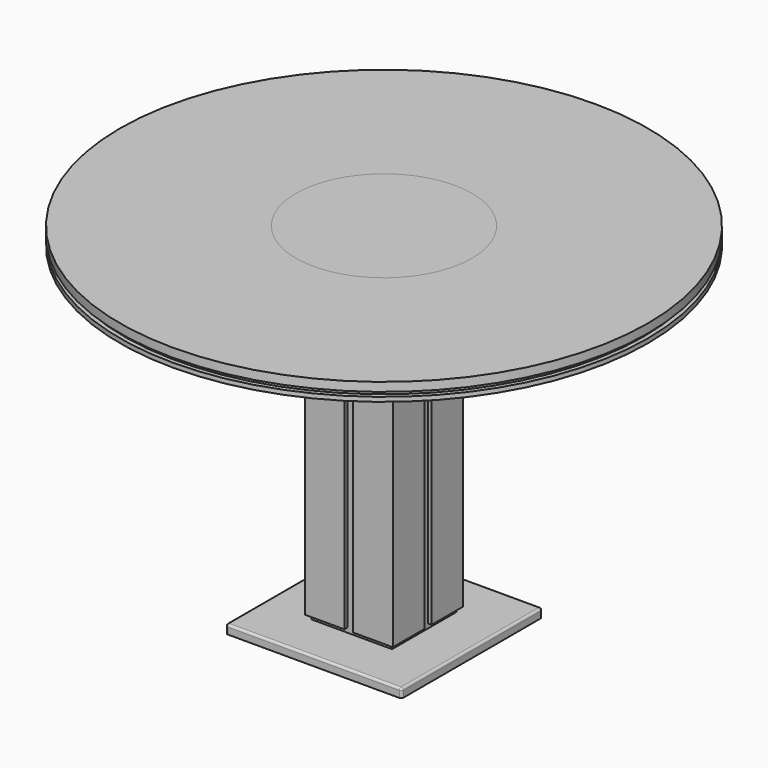
from build123d import *

# Parameters (mm, degrees)
F1_START  = 30
F1_DEPTH  = 720
F2_START  = 30
F0_W      = 20
F0_H      = 8.1586758983
F2_DEPTH  = 720
F0_W_2    = 8.1586758983
F0_H_2    = 20
F3_START  = 20
F3_DEPTH  = 10
F4_START  = 750
F4_DEPTH  = 10
F0_W_3    = 400
F0_H_3    = 400
F5_DEPTH  = 20
F7_START  = 20
F6_R      = 600
F6_R_2    = 590
F6_R_3    = 200
F7_DEPTH  = 20
F8_START  = 10
F6_W      = 183.6826482035
F6_H      = 183.6826482035
F8_DEPTH  = 10
F9_DEPTH  = 10
F10_START = 30
F10_DEPTH = 10
F11_DEPTH = 10
F12_R     = 5


with BuildPart() as f1:
    # F0 (on Top) → F1 (new body)
    with BuildSketch(Plane.XY.offset(F1_START)):
        Polygon((10, 83.6826482035), (-10, 83.6826482035), (-10, 91.8413241017), (-91.8413241017, 91.8413241017), (-91.8413241017, 10), (-83.6826482035, 10), (-83.6826482035, -10), (-91.8413241017, -10), (-91.8413241017, -91.8413241017), (-10, -91.8413241017), (-10, -83.6826482035), (10, -83.6826482035), (10, -91.8413241017), (91.8413241017, -91.8413241017), (91.8413241017, -10), (83.6826482035, -10), (83.6826482035, 10), (91.8413241017, 10), (91.8413241017, 91.8413241017), (10, 91.8413241017), align=None)
        Polygon((-91.8413241017, 91.8413241017), (-10, 91.8413241017), (-10, 100), (-100, 100), (-100, 10), (-91.8413241017, 10), align=None)
        Polygon((-91.8413241017, -91.8413241017), (-91.8413241017, -10), (-100, -10), (-100, -100), (-10, -100), (-10, -91.8413241017), align=None)
        Polygon((100, -10), (91.8413241017, -10), (91.8413241017, -91.8413241017), (10, -91.8413241017), (10, -100), (100, -100), align=None)
        Polygon((10, 100), (10, 91.8413241017), (91.8413241017, 91.8413241017), (91.8413241017, 10), (100, 10), (100, 100), align=None)
    extrude(amount=F1_DEPTH)


with BuildPart() as f2:
    # F0 (on Top) → F2 (new body)
    with BuildSketch(Plane.XY.offset(F2_START)):
        with Locations((0, -87.7619861526)):
            Rectangle(F0_W, F0_H)
    extrude(amount=F2_DEPTH)



with BuildPart() as f2b:
    # F0 (on Top) → F2, piece 2 (new body)
    with BuildSketch(Plane.XY.offset(F2_START)):
        with Locations((87.7619861526, 0)):
            Rectangle(F0_W_2, F0_H_2)
    extrude(amount=F2_DEPTH)


with BuildPart() as f2c:
    # F0 (on Top) → F2, piece 3 (new body)
    with BuildSketch(Plane.XY.offset(F2_START)):
        with Locations((0, 87.7619861526)):
            Rectangle(F0_W, F0_H)
    extrude(amount=F2_DEPTH)


with BuildPart() as f2d:
    # F0 (on Top) → F2, piece 4 (new body)
    with BuildSketch(Plane.XY.offset(F2_START)):
        with Locations((-87.7619861526, 0)):
            Rectangle(F0_W_2, F0_H_2)
    extrude(amount=F2_DEPTH)


with BuildPart() as f2_1:
    add(f2.part)

    add(f2b.part)  # F3 merges F2b

    add(f2c.part)  # F3 merges F2c

    add(f2d.part)  # F3 merges F2d
    # F0 (on Top) → F3 (join)
    with BuildSketch(Plane.XY.offset(F3_START)):
        Polygon((10, 83.6826482035), (-10, 83.6826482035), (-10, 91.8413241017), (-91.8413241017, 91.8413241017), (-91.8413241017, 10), (-83.6826482035, 10), (-83.6826482035, -10), (-91.8413241017, -10), (-91.8413241017, -91.8413241017), (-10, -91.8413241017), (-10, -83.6826482035), (10, -83.6826482035), (10, -91.8413241017), (91.8413241017, -91.8413241017), (91.8413241017, -10), (83.6826482035, -10), (83.6826482035, 10), (91.8413241017, 10), (91.8413241017, 91.8413241017), (10, 91.8413241017), align=None)
        with Locations((0, -87.7619861526)):
            Rectangle(F0_W, F0_H)
        with Locations((87.7619861526, 0)):
            Rectangle(F0_W_2, F0_H_2)
        with Locations((0, 87.7619861526)):
            Rectangle(F0_W, F0_H)
        with Locations((-87.7619861526, 0)):
            Rectangle(F0_W_2, F0_H_2)
    extrude(amount=F3_DEPTH)

    # F0 (on Top) → F4 (join)
    with BuildSketch(Plane.XY.offset(F4_START)):
        Polygon((10, 83.6826482035), (-10, 83.6826482035), (-10, 91.8413241017), (-91.8413241017, 91.8413241017), (-91.8413241017, 10), (-83.6826482035, 10), (-83.6826482035, -10), (-91.8413241017, -10), (-91.8413241017, -91.8413241017), (-10, -91.8413241017), (-10, -83.6826482035), (10, -83.6826482035), (10, -91.8413241017), (91.8413241017, -91.8413241017), (91.8413241017, -10), (83.6826482035, -10), (83.6826482035, 10), (91.8413241017, 10), (91.8413241017, 91.8413241017), (10, 91.8413241017), align=None)
        with Locations((0, 87.7619861526)):
            Rectangle(F0_W, F0_H)
        with Locations((-87.7619861526, 0)):
            Rectangle(F0_W_2, F0_H_2)
        with Locations((0, -87.7619861526)):
            Rectangle(F0_W, F0_H)
        with Locations((87.7619861526, 0)):
            Rectangle(F0_W_2, F0_H_2)
    extrude(amount=F4_DEPTH)

    # F0 (on Top) → F5 (join)
    with BuildSketch(Plane.XY):
        Rectangle(F0_W_3, F0_H_3)
        Polygon((-10, 100), (-10, 91.8413241017), (10, 91.8413241017), (10, 100), (100, 100), (100, 10), (91.8413241017, 10), (91.8413241017, -10), (100, -10), (100, -100), (10, -100), (10, -91.8413241017), (-10, -91.8413241017), (-10, -100), (-100, -100), (-100, -10), (-91.8413241017, -10), (-91.8413241017, 10), (-100, 10), (-100, 100), align=None, mode=Mode.SUBTRACT)
        Polygon((-91.8413241017, 91.8413241017), (-10, 91.8413241017), (-10, 100), (-100, 100), (-100, 10), (-91.8413241017, 10), align=None)
        Polygon((10, 100), (10, 91.8413241017), (91.8413241017, 91.8413241017), (91.8413241017, 10), (100, 10), (100, 100), align=None)
        Polygon((100, -10), (91.8413241017, -10), (91.8413241017, -91.8413241017), (10, -91.8413241017), (10, -100), (100, -100), align=None)
        Polygon((-91.8413241017, -91.8413241017), (-91.8413241017, -10), (-100, -10), (-100, -100), (-10, -100), (-10, -91.8413241017), align=None)
        with Locations((-87.7619861526, 0)):
            Rectangle(F0_W_2, F0_H_2)
        with Locations((0, 87.7619861526)):
            Rectangle(F0_W, F0_H)
        with Locations((87.7619861526, 0)):
            Rectangle(F0_W_2, F0_H_2)
        with Locations((0, -87.7619861526)):
            Rectangle(F0_W, F0_H)
        Polygon((10, 83.6826482035), (-10, 83.6826482035), (-10, 91.8413241017), (-91.8413241017, 91.8413241017), (-91.8413241017, 10), (-83.6826482035, 10), (-83.6826482035, -10), (-91.8413241017, -10), (-91.8413241017, -91.8413241017), (-10, -91.8413241017), (-10, -83.6826482035), (10, -83.6826482035), (10, -91.8413241017), (91.8413241017, -91.8413241017), (91.8413241017, -10), (83.6826482035, -10), (83.6826482035, 10), (91.8413241017, 10), (91.8413241017, 91.8413241017), (10, 91.8413241017), align=None)
    extrude(amount=F5_DEPTH)

    # F12
    f12_edges = [f2_1.edges().sort_by_distance(p)[0] for p in [
        (0, -200, 20),
        (-200, 0, 20),
        (0, 200, 20),
        (200, 0, 20),
        (200, 200, 10),
        (-200, 200, 10),
        (-200, -200, 10),
        (200, -200, 10),
    ]]
    fillet(f12_edges, radius=F12_R)


with BuildPart() as f7:
    # F6 (on face) → F7 (new body)
    with BuildSketch(Plane.XY.offset(760).offset(F7_START)):
        Circle(F6_R)
        Circle(F6_R_2, mode=Mode.SUBTRACT)
        Circle(F6_R_2)
        Circle(F6_R_3, mode=Mode.SUBTRACT)
    extrude(amount=F7_DEPTH)


with BuildPart() as f8:
    # F6 (on face) → F8 (new body)
    with BuildSketch(Plane.XY.offset(760).offset(F8_START)):
        Circle(F6_R_2)
        Circle(F6_R_3, mode=Mode.SUBTRACT)
        Circle(F6_R_3)
        Rectangle(F6_W, F6_H, mode=Mode.SUBTRACT)
    extrude(amount=F8_DEPTH)


with BuildPart() as f9:
    # F6 (on face) → F9 (new body)
    with BuildSketch(Plane.XY.offset(760)):
        Circle(F6_R)
        Circle(F6_R_2, mode=Mode.SUBTRACT)
        Circle(F6_R_2)
        Circle(F6_R_3, mode=Mode.SUBTRACT)
        Circle(F6_R_3)
        Rectangle(F6_W, F6_H, mode=Mode.SUBTRACT)
    extrude(amount=F9_DEPTH)


with BuildPart() as f10:
    # F6 (on face) → F10 (new body)
    with BuildSketch(Plane.XY.offset(760).offset(F10_START)):
        Circle(F6_R_3)
        Rectangle(F6_W, F6_H, mode=Mode.SUBTRACT)
        Rectangle(F6_W, F6_H)
    extrude(amount=F10_DEPTH)


with BuildPart() as f11:
    # F11 (new): a face of the model
    f11_faces = [f10.part.faces().sort_by_distance(p)[0] for p in [
        (0, 0, 790),
    ]]
    extrude(f11_faces, amount=F11_DEPTH)


solid = Compound([f1.part, f2_1.part, f7.part, f8.part, f9.part, f10.part, f11.part])
